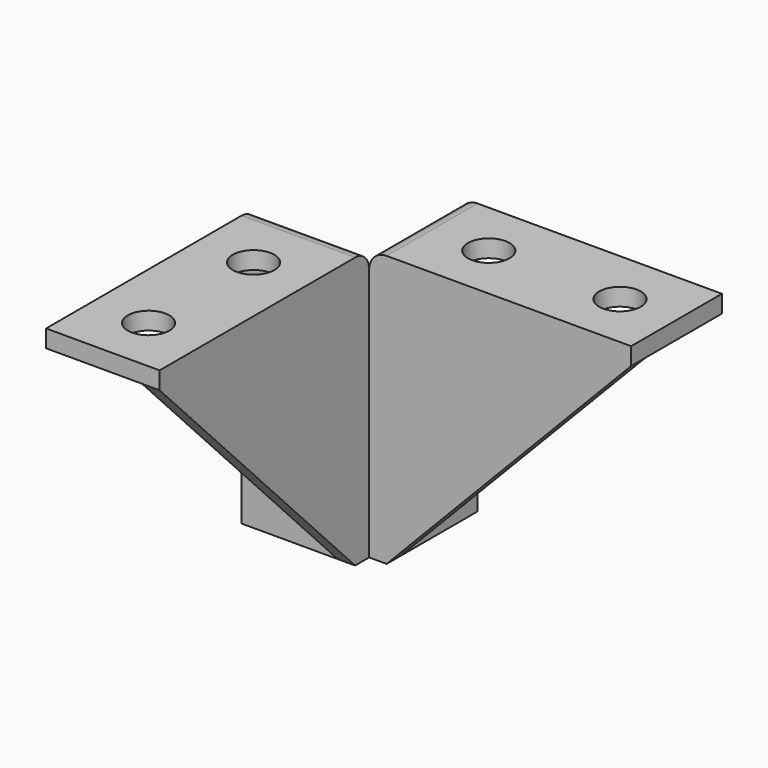
from build123d import *

# Parameters (mm, degrees)
F1_DEPTH     = 41.1988
F3_DEPTH     = 41.1988
F4_T1_DEPTH  = 72.9488
F5_R         = 6.35
F14_D        = 15.08252
F14_ON_F9_D  = 15.08252
F14_ON_F11_D = 15.08252
F14_ON_F13_D = 15.08252
F17_DEPTH    = 88.9
F20_DEPTH    = 6.35
F23_DEPTH    = 6.35


# Not quite as in the source:
# - a fillet or chamfer that OpenCascade refuses, or shapes differently, is made with other operations: its cross-section is extruded or revolved along the edge and cut away or added


with BuildPart() as f1:
    # F0 (on Right) → F1 (new body)
    with BuildSketch(Plane.YZ):
        Polygon((0, 98.425), (-95.0722, 98.425), (-95.0722, 92.075), (-6.35, 92.075), (-6.35, 0), (0, 0), align=None)
    extrude(amount=-F1_DEPTH)

    # F2 (on Front) → F3 (join)
    with BuildSketch(Plane.XZ):
        Polygon((95.0722, 92.075), (95.0722, 98.425), (0, 98.425), (0, 0), (6.35, 0), (6.35, 92.075), align=None)
    extrude(amount=-F3_DEPTH)

    # F4: fillet of radius 6.35 on 1 edges, made by hand

    # F4_s2 → F4_t1 (cut)
    with BuildSketch(Plane.YZ.offset(-57.0738)):
        with BuildLine():
            ThreePointArc((-6.35, 98.425), (-1.8598719395, 96.5651280605), (0, 92.075))
            Line((0, 92.075), (0, 98.425))
            Line((0, 98.425), (-6.35, 98.425))
        make_face()
    extrude(amount=F4_T1_DEPTH, mode=Mode.SUBTRACT)

    # F5
    f5_edges = [f1.edges().sort_by_distance(p)[0] for p in [
        (0, 20.5994, 98.425),
    ]]
    fillet(f5_edges, radius=F5_R)

    # F14 (through all)
    with Locations(Plane(origin=(0, 0, 0), x_dir=(-1, 0, 0), z_dir=(0, 1, 0))):
        with Locations((20.5994, 23.84425), (20.5994, 71.46925)):
            Hole(F14_D / 2)

    # F14 on F9 (through all)
    with Locations(Plane.XY.offset(98.425)):
        with Locations((-20.5994, -26.68524), (-20.5994, -74.31024)):
            Hole(F14_ON_F9_D / 2)

    # F14 on F11 (through all)
    with Locations(Plane(origin=(0, 0, 0), x_dir=(0, -1, 0), z_dir=(-1, 0, 0))):
        with Locations((-20.5994, 23.84425), (-20.5994, 71.46925)):
            Hole(F14_ON_F11_D / 2)

    # F14 on F13 (through all)
    with Locations(Plane.XY.offset(98.425)):
        with Locations((26.9367, 20.5994), (74.5617, 20.5994)):
            Hole(F14_ON_F13_D / 2)

    # F19 (on offset) → F20 (join)
    with BuildSketch(Plane.YZ):
        Polygon((-6.35, 0), (-6.35, 92.075), (-95.0722, 92.075), align=None)
    extrude(amount=-F20_DEPTH)

    # F22 (on offset) → F23 (join)
    with BuildSketch(Plane.XZ):
        Polygon((95.0722, 92.075), (6.35, 92.075), (6.35, 0), align=None)
    extrude(amount=-F23_DEPTH)


with BuildPart() as f17:
    # F16 (on offset) → F17 (new body)
    with BuildSketch(Plane(origin=(0, 0, 0), x_dir=(1, 0, 0), z_dir=(0, 0, -1))):
        with BuildLine():
            ThreePointArc((-6.35, 0), (-1.8598719395, -1.8598719395), (0, -6.35))
            Line((0, -6.35), (0, 0))
            Line((0, 0), (-6.35, 0))
        make_face()
    extrude(amount=-F17_DEPTH)


solid = Compound([f1.part, f17.part])
